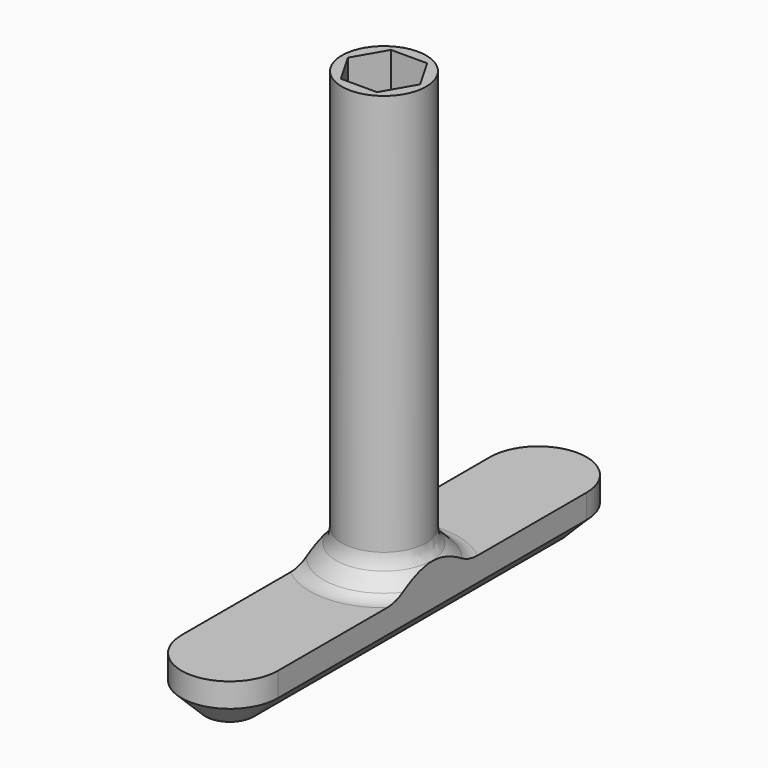
from build123d import *

# Parameters (mm, degrees)
F0_R     = 8.75
F1_DEPTH = 90
F3_DEPTH = 10
F5_R     = 4
F6_SIZE  = 5


# Not quite as in the source:
# - a fillet or chamfer that OpenCascade refuses, or shapes differently, is made with other operations: its cross-section is extruded or revolved along the edge and cut away or added


with BuildPart() as f1:
    # F0 (on Top) → F1 (new body)
    with BuildSketch(Plane.XY):
        Circle(F0_R)
        Polygon((3.75, 6.4951905284), (7.5, 0), (3.75, -6.4951905284), (-3.75, -6.4951905284), (-7.5, 0), (-3.75, 6.4951905284), align=None, mode=Mode.SUBTRACT)
    extrude(amount=F1_DEPTH)

    # F2 (on Top) → F3 (join)
    with BuildSketch(Plane.XY):
        with BuildLine():
            ThreePointArc((10, 40), (0, 50), (-10, 40))
            Line((-10, 40), (-10, 0))
            Line((-10, 0), (-10, -40))
            ThreePointArc((-10, -40), (0, -50), (10, -40))
            Line((10, -40), (10, 0))
            Line((10, 0), (10, 40))
        make_face()
    extrude(amount=-F3_DEPTH)

    # F4: chamfer of 5 on 1 edges, made by hand


with BuildPart() as f4_tool2:
    # F4_s3 → F4_t4 (revolve)
    with BuildSketch(Plane.XZ):
        Polygon((13.75, 0), (8.75, 5), (8.75, 0), align=None)
    revolve(axis=Axis((0, 0, 0), (0, 0, 1)))

    split(bisect_by=Plane.YZ.offset(10), keep=Keep.BOTTOM)

    split(bisect_by=Plane.YZ.offset(-10), keep=Keep.TOP)


with BuildPart() as f1_1:
    add(f1.part)

    # F4_t1: union F4_tool2
    add(f4_tool2.part)

    # F5
    f5_edges = [f1_1.edges().sort_by_distance(p)[0] for p in [
        (0, -13.75, 0),
        (0, 13.75, 0),
        (-8.75, 0, 5),
    ]]
    fillet(f5_edges, radius=F5_R)

    # F6
    f6_edges = [f1_1.edges().sort_by_distance(p)[0] for p in [
        (10, 0, -10),
    ]]
    chamfer(f6_edges, length=F6_SIZE)


solid = f1_1.part
